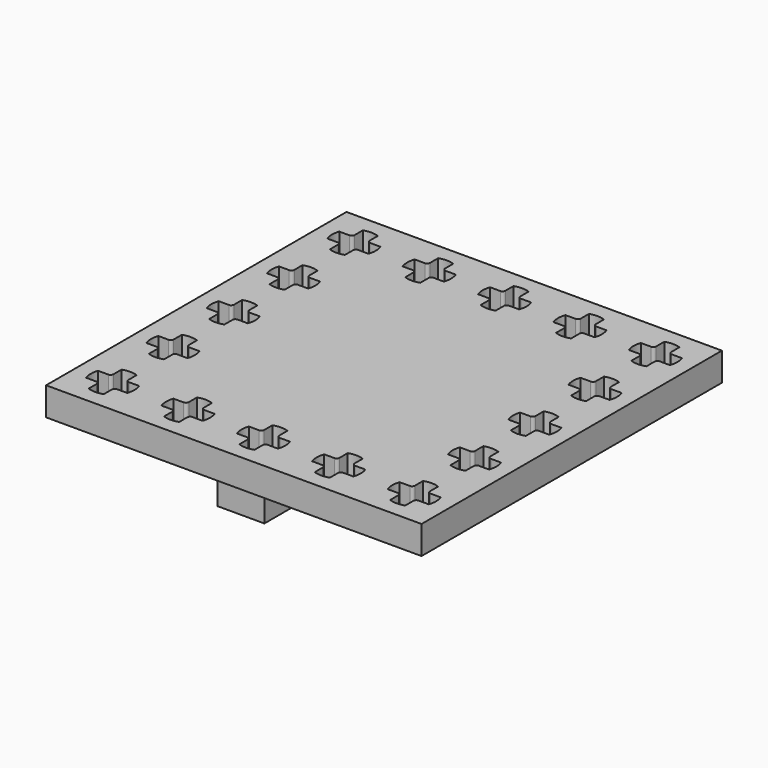
from build123d import *

# Parameters (mm, degrees)
F0_W     = 39.85
F0_H     = 39.85
F1_DEPTH = 6
F3_W     = 39.85
F3_H     = 39.85
F4_DEPTH = 3


# Not quite as in the source:
# - a feature names something its author has since deleted; it is built from what else it names


with BuildPart() as f1:
    # F0 (on Top) → F1 (new body)
    with BuildSketch(Plane.XY):
        Rectangle(F0_W, F0_H)
        with BuildLine():
            ThreePointArc((-16.8, -13.8169688504), (-16, -13.675), (-15.2, -13.8169688504))
            Line((-15.2, -13.8169688504), (-15.2, -14.9))
            ThreePointArc((-15.2, -14.9), (-15.1121320344, -15.1121320344), (-14.9, -15.2))
            Line((-14.9, -15.2), (-13.8169688504, -15.2))
            ThreePointArc((-13.8169688504, -15.2), (-13.675, -16), (-13.8169688504, -16.8))
            Line((-13.8169688504, -16.8), (-14.9, -16.8))
            ThreePointArc((-14.9, -16.8), (-15.1121320344, -16.8878679656), (-15.2, -17.1))
            Line((-15.2, -17.1), (-15.2, -18.1830311496))
            ThreePointArc((-15.2, -18.1830311496), (-16, -18.325), (-16.8, -18.1830311496))
            Line((-16.8, -18.1830311496), (-16.8, -17.1))
            ThreePointArc((-16.8, -17.1), (-16.8878679656, -16.8878679656), (-17.1, -16.8))
            Line((-17.1, -16.8), (-18.1830311496, -16.8))
            ThreePointArc((-18.1830311496, -16.8), (-18.325, -16), (-18.1830311496, -15.2))
            Line((-18.1830311496, -15.2), (-17.1, -15.2))
            ThreePointArc((-17.1, -15.2), (-16.8878679656, -15.1121320344), (-16.8, -14.9))
            Line((-16.8, -14.9), (-16.8, -13.8169688504))
        make_face(mode=Mode.SUBTRACT)
        with BuildLine():
            ThreePointArc((-8.8, -13.8169688504), (-8, -13.675), (-7.2, -13.8169688504))
            Line((-7.2, -13.8169688504), (-7.2, -14.9))
            ThreePointArc((-7.2, -14.9), (-7.1121320344, -15.1121320344), (-6.9, -15.2))
            Line((-6.9, -15.2), (-5.8169688504, -15.2))
            ThreePointArc((-5.8169688504, -15.2), (-5.675, -16), (-5.8169688504, -16.8))
            Line((-5.8169688504, -16.8), (-6.9, -16.8))
            ThreePointArc((-6.9, -16.8), (-7.1121320344, -16.8878679656), (-7.2, -17.1))
            Line((-7.2, -17.1), (-7.2, -18.1830311496))
            ThreePointArc((-7.2, -18.1830311496), (-8, -18.325), (-8.8, -18.1830311496))
            Line((-8.8, -18.1830311496), (-8.8, -17.1))
            ThreePointArc((-8.8, -17.1), (-8.8878679656, -16.8878679656), (-9.1, -16.8))
            Line((-9.1, -16.8), (-10.1830311496, -16.8))
            ThreePointArc((-10.1830311496, -16.8), (-10.325, -16), (-10.1830311496, -15.2))
            Line((-10.1830311496, -15.2), (-9.1, -15.2))
            ThreePointArc((-9.1, -15.2), (-8.8878679656, -15.1121320344), (-8.8, -14.9))
            Line((-8.8, -14.9), (-8.8, -13.8169688504))
        make_face(mode=Mode.SUBTRACT)
        with BuildLine():
            ThreePointArc((-16.8, -5.8169688504), (-16, -5.675), (-15.2, -5.8169688504))
            Line((-15.2, -5.8169688504), (-15.2, -6.9))
            ThreePointArc((-15.2, -6.9), (-15.1121320344, -7.1121320344), (-14.9, -7.2))
            Line((-14.9, -7.2), (-13.8169688504, -7.2))
            ThreePointArc((-13.8169688504, -7.2), (-13.675, -8), (-13.8169688504, -8.8))
            Line((-13.8169688504, -8.8), (-14.9, -8.8))
            ThreePointArc((-14.9, -8.8), (-15.1121320344, -8.8878679656), (-15.2, -9.1))
            Line((-15.2, -9.1), (-15.2, -10.1830311496))
            ThreePointArc((-15.2, -10.1830311496), (-16, -10.325), (-16.8, -10.1830311496))
            Line((-16.8, -10.1830311496), (-16.8, -9.1))
            ThreePointArc((-16.8, -9.1), (-16.8878679656, -8.8878679656), (-17.1, -8.8))
            Line((-17.1, -8.8), (-18.1830311496, -8.8))
            ThreePointArc((-18.1830311496, -8.8), (-18.325, -8), (-18.1830311496, -7.2))
            Line((-18.1830311496, -7.2), (-17.1, -7.2))
            ThreePointArc((-17.1, -7.2), (-16.8878679656, -7.1121320344), (-16.8, -6.9))
            Line((-16.8, -6.9), (-16.8, -5.8169688504))
        make_face(mode=Mode.SUBTRACT)
        with BuildLine():
            ThreePointArc((-8.8, -5.8169688504), (-8, -5.675), (-7.2, -5.8169688504))
            Line((-7.2, -5.8169688504), (-7.2, -6.9))
            ThreePointArc((-7.2, -6.9), (-7.1121320344, -7.1121320344), (-6.9, -7.2))
            Line((-6.9, -7.2), (-5.8169688504, -7.2))
            ThreePointArc((-5.8169688504, -7.2), (-5.675, -8), (-5.8169688504, -8.8))
            Line((-5.8169688504, -8.8), (-6.9, -8.8))
            ThreePointArc((-6.9, -8.8), (-7.1121320344, -8.8878679656), (-7.2, -9.1))
            Line((-7.2, -9.1), (-7.2, -10.1830311496))
            ThreePointArc((-7.2, -10.1830311496), (-8, -10.325), (-8.8, -10.1830311496))
            Line((-8.8, -10.1830311496), (-8.8, -9.1))
            ThreePointArc((-8.8, -9.1), (-8.8878679656, -8.8878679656), (-9.1, -8.8))
            Line((-9.1, -8.8), (-10.1830311496, -8.8))
            ThreePointArc((-10.1830311496, -8.8), (-10.325, -8), (-10.1830311496, -7.2))
            Line((-10.1830311496, -7.2), (-9.1, -7.2))
            ThreePointArc((-9.1, -7.2), (-8.8878679656, -7.1121320344), (-8.8, -6.9))
            Line((-8.8, -6.9), (-8.8, -5.8169688504))
        make_face(mode=Mode.SUBTRACT)
        with BuildLine():
            ThreePointArc((-0.8, -13.8169688504), (0, -13.675), (0.8, -13.8169688504))
            Line((0.8, -13.8169688504), (0.8, -14.9))
            ThreePointArc((0.8, -14.9), (0.8878679656, -15.1121320344), (1.1, -15.2))
            Line((1.1, -15.2), (2.1830311496, -15.2))
            ThreePointArc((2.1830311496, -15.2), (2.325, -16), (2.1830311496, -16.8))
            Line((2.1830311496, -16.8), (1.1, -16.8))
            ThreePointArc((1.1, -16.8), (0.8878679656, -16.8878679656), (0.8, -17.1))
            Line((0.8, -17.1), (0.8, -18.1830311496))
            ThreePointArc((0.8, -18.1830311496), (0, -18.325), (-0.8, -18.1830311496))
            Line((-0.8, -18.1830311496), (-0.8, -17.1))
            ThreePointArc((-0.8, -17.1), (-0.8878679656, -16.8878679656), (-1.1, -16.8))
            Line((-1.1, -16.8), (-2.1830311496, -16.8))
            ThreePointArc((-2.1830311496, -16.8), (-2.325, -16), (-2.1830311496, -15.2))
            Line((-2.1830311496, -15.2), (-1.1, -15.2))
            ThreePointArc((-1.1, -15.2), (-0.8878679656, -15.1121320344), (-0.8, -14.9))
            Line((-0.8, -14.9), (-0.8, -13.8169688504))
        make_face(mode=Mode.SUBTRACT)
        with BuildLine():
            ThreePointArc((7.2, -13.8169688504), (8, -13.675), (8.8, -13.8169688504))
            Line((8.8, -13.8169688504), (8.8, -14.9))
            ThreePointArc((8.8, -14.9), (8.8878679656, -15.1121320344), (9.1, -15.2))
            Line((9.1, -15.2), (10.1830311496, -15.2))
            ThreePointArc((10.1830311496, -15.2), (10.325, -16), (10.1830311496, -16.8))
            Line((10.1830311496, -16.8), (9.1, -16.8))
            ThreePointArc((9.1, -16.8), (8.8878679656, -16.8878679656), (8.8, -17.1))
            Line((8.8, -17.1), (8.8, -18.1830311496))
            ThreePointArc((8.8, -18.1830311496), (8, -18.325), (7.2, -18.1830311496))
            Line((7.2, -18.1830311496), (7.2, -17.1))
            ThreePointArc((7.2, -17.1), (7.1121320344, -16.8878679656), (6.9, -16.8))
            Line((6.9, -16.8), (5.8169688504, -16.8))
            ThreePointArc((5.8169688504, -16.8), (5.675, -16), (5.8169688504, -15.2))
            Line((5.8169688504, -15.2), (6.9, -15.2))
            ThreePointArc((6.9, -15.2), (7.1121320344, -15.1121320344), (7.2, -14.9))
            Line((7.2, -14.9), (7.2, -13.8169688504))
        make_face(mode=Mode.SUBTRACT)
        with BuildLine():
            ThreePointArc((15.2, -13.8169688504), (16, -13.675), (16.8, -13.8169688504))
            Line((16.8, -13.8169688504), (16.8, -14.9))
            ThreePointArc((16.8, -14.9), (16.8878679656, -15.1121320344), (17.1, -15.2))
            Line((17.1, -15.2), (18.1830311496, -15.2))
            ThreePointArc((18.1830311496, -15.2), (18.325, -16), (18.1830311496, -16.8))
            Line((18.1830311496, -16.8), (17.1, -16.8))
            ThreePointArc((17.1, -16.8), (16.8878679656, -16.8878679656), (16.8, -17.1))
            Line((16.8, -17.1), (16.8, -18.1830311496))
            ThreePointArc((16.8, -18.1830311496), (16, -18.325), (15.2, -18.1830311496))
            Line((15.2, -18.1830311496), (15.2, -17.1))
            ThreePointArc((15.2, -17.1), (15.1121320344, -16.8878679656), (14.9, -16.8))
            Line((14.9, -16.8), (13.8169688504, -16.8))
            ThreePointArc((13.8169688504, -16.8), (13.675, -16), (13.8169688504, -15.2))
            Line((13.8169688504, -15.2), (14.9, -15.2))
            ThreePointArc((14.9, -15.2), (15.1121320344, -15.1121320344), (15.2, -14.9))
            Line((15.2, -14.9), (15.2, -13.8169688504))
        make_face(mode=Mode.SUBTRACT)
        with BuildLine():
            ThreePointArc((-0.8, -5.8169688504), (0, -5.675), (0.8, -5.8169688504))
            Line((0.8, -5.8169688504), (0.8, -6.9))
            ThreePointArc((0.8, -6.9), (0.8878679656, -7.1121320344), (1.1, -7.2))
            Line((1.1, -7.2), (2.1830311496, -7.2))
            ThreePointArc((2.1830311496, -7.2), (2.325, -8), (2.1830311496, -8.8))
            Line((2.1830311496, -8.8), (1.1, -8.8))
            ThreePointArc((1.1, -8.8), (0.8878679656, -8.8878679656), (0.8, -9.1))
            Line((0.8, -9.1), (0.8, -10.1830311496))
            ThreePointArc((0.8, -10.1830311496), (0, -10.325), (-0.8, -10.1830311496))
            Line((-0.8, -10.1830311496), (-0.8, -9.1))
            ThreePointArc((-0.8, -9.1), (-0.8878679656, -8.8878679656), (-1.1, -8.8))
            Line((-1.1, -8.8), (-2.1830311496, -8.8))
            ThreePointArc((-2.1830311496, -8.8), (-2.325, -8), (-2.1830311496, -7.2))
            Line((-2.1830311496, -7.2), (-1.1, -7.2))
            ThreePointArc((-1.1, -7.2), (-0.8878679656, -7.1121320344), (-0.8, -6.9))
            Line((-0.8, -6.9), (-0.8, -5.8169688504))
        make_face(mode=Mode.SUBTRACT)
        with BuildLine():
            ThreePointArc((7.2, -5.8169688504), (8, -5.675), (8.8, -5.8169688504))
            Line((8.8, -5.8169688504), (8.8, -6.9))
            ThreePointArc((8.8, -6.9), (8.8878679656, -7.1121320344), (9.1, -7.2))
            Line((9.1, -7.2), (10.1830311496, -7.2))
            ThreePointArc((10.1830311496, -7.2), (10.325, -8), (10.1830311496, -8.8))
            Line((10.1830311496, -8.8), (9.1, -8.8))
            ThreePointArc((9.1, -8.8), (8.8878679656, -8.8878679656), (8.8, -9.1))
            Line((8.8, -9.1), (8.8, -10.1830311496))
            ThreePointArc((8.8, -10.1830311496), (8, -10.325), (7.2, -10.1830311496))
            Line((7.2, -10.1830311496), (7.2, -9.1))
            ThreePointArc((7.2, -9.1), (7.1121320344, -8.8878679656), (6.9, -8.8))
            Line((6.9, -8.8), (5.8169688504, -8.8))
            ThreePointArc((5.8169688504, -8.8), (5.675, -8), (5.8169688504, -7.2))
            Line((5.8169688504, -7.2), (6.9, -7.2))
            ThreePointArc((6.9, -7.2), (7.1121320344, -7.1121320344), (7.2, -6.9))
            Line((7.2, -6.9), (7.2, -5.8169688504))
        make_face(mode=Mode.SUBTRACT)
        with BuildLine():
            ThreePointArc((15.2, -5.8169688504), (16, -5.675), (16.8, -5.8169688504))
            Line((16.8, -5.8169688504), (16.8, -6.9))
            ThreePointArc((16.8, -6.9), (16.8878679656, -7.1121320344), (17.1, -7.2))
            Line((17.1, -7.2), (18.1830311496, -7.2))
            ThreePointArc((18.1830311496, -7.2), (18.325, -8), (18.1830311496, -8.8))
            Line((18.1830311496, -8.8), (17.1, -8.8))
            ThreePointArc((17.1, -8.8), (16.8878679656, -8.8878679656), (16.8, -9.1))
            Line((16.8, -9.1), (16.8, -10.1830311496))
            ThreePointArc((16.8, -10.1830311496), (16, -10.325), (15.2, -10.1830311496))
            Line((15.2, -10.1830311496), (15.2, -9.1))
            ThreePointArc((15.2, -9.1), (15.1121320344, -8.8878679656), (14.9, -8.8))
            Line((14.9, -8.8), (13.8169688504, -8.8))
            ThreePointArc((13.8169688504, -8.8), (13.675, -8), (13.8169688504, -7.2))
            Line((13.8169688504, -7.2), (14.9, -7.2))
            ThreePointArc((14.9, -7.2), (15.1121320344, -7.1121320344), (15.2, -6.9))
            Line((15.2, -6.9), (15.2, -5.8169688504))
        make_face(mode=Mode.SUBTRACT)
        with BuildLine():
            ThreePointArc((-16.8, 2.1830311496), (-16, 2.325), (-15.2, 2.1830311496))
            Line((-15.2, 2.1830311496), (-15.2, 1.1))
            ThreePointArc((-15.2, 1.1), (-15.1121320344, 0.8878679656), (-14.9, 0.8))
            Line((-14.9, 0.8), (-13.8169688504, 0.8))
            ThreePointArc((-13.8169688504, 0.8), (-13.675, 0), (-13.8169688504, -0.8))
            Line((-13.8169688504, -0.8), (-14.9, -0.8))
            ThreePointArc((-14.9, -0.8), (-15.1121320344, -0.8878679656), (-15.2, -1.1))
            Line((-15.2, -1.1), (-15.2, -2.1830311496))
            ThreePointArc((-15.2, -2.1830311496), (-16, -2.325), (-16.8, -2.1830311496))
            Line((-16.8, -2.1830311496), (-16.8, -1.1))
            ThreePointArc((-16.8, -1.1), (-16.8878679656, -0.8878679656), (-17.1, -0.8))
            Line((-17.1, -0.8), (-18.1830311496, -0.8))
            ThreePointArc((-18.1830311496, -0.8), (-18.325, 0), (-18.1830311496, 0.8))
            Line((-18.1830311496, 0.8), (-17.1, 0.8))
            ThreePointArc((-17.1, 0.8), (-16.8878679656, 0.8878679656), (-16.8, 1.1))
            Line((-16.8, 1.1), (-16.8, 2.1830311496))
        make_face(mode=Mode.SUBTRACT)
        with BuildLine():
            ThreePointArc((-16.8, 10.1830311496), (-16, 10.325), (-15.2, 10.1830311496))
            Line((-15.2, 10.1830311496), (-15.2, 9.1))
            ThreePointArc((-15.2, 9.1), (-15.1121320344, 8.8878679656), (-14.9, 8.8))
            Line((-14.9, 8.8), (-13.8169688504, 8.8))
            ThreePointArc((-13.8169688504, 8.8), (-13.675, 8), (-13.8169688504, 7.2))
            Line((-13.8169688504, 7.2), (-14.9, 7.2))
            ThreePointArc((-14.9, 7.2), (-15.1121320344, 7.1121320344), (-15.2, 6.9))
            Line((-15.2, 6.9), (-15.2, 5.8169688504))
            ThreePointArc((-15.2, 5.8169688504), (-16, 5.675), (-16.8, 5.8169688504))
            Line((-16.8, 5.8169688504), (-16.8, 6.9))
            ThreePointArc((-16.8, 6.9), (-16.8878679656, 7.1121320344), (-17.1, 7.2))
            Line((-17.1, 7.2), (-18.1830311496, 7.2))
            ThreePointArc((-18.1830311496, 7.2), (-18.325, 8), (-18.1830311496, 8.8))
            Line((-18.1830311496, 8.8), (-17.1, 8.8))
            ThreePointArc((-17.1, 8.8), (-16.8878679656, 8.8878679656), (-16.8, 9.1))
            Line((-16.8, 9.1), (-16.8, 10.1830311496))
        make_face(mode=Mode.SUBTRACT)
        with BuildLine():
            ThreePointArc((-8.8, 2.1830311496), (-8, 2.325), (-7.2, 2.1830311496))
            Line((-7.2, 2.1830311496), (-7.2, 1.1))
            ThreePointArc((-7.2, 1.1), (-7.1121320344, 0.8878679656), (-6.9, 0.8))
            Line((-6.9, 0.8), (-5.8169688504, 0.8))
            ThreePointArc((-5.8169688504, 0.8), (-5.675, 0), (-5.8169688504, -0.8))
            Line((-5.8169688504, -0.8), (-6.9, -0.8))
            ThreePointArc((-6.9, -0.8), (-7.1121320344, -0.8878679656), (-7.2, -1.1))
            Line((-7.2, -1.1), (-7.2, -2.1830311496))
            ThreePointArc((-7.2, -2.1830311496), (-8, -2.325), (-8.8, -2.1830311496))
            Line((-8.8, -2.1830311496), (-8.8, -1.1))
            ThreePointArc((-8.8, -1.1), (-8.8878679656, -0.8878679656), (-9.1, -0.8))
            Line((-9.1, -0.8), (-10.1830311496, -0.8))
            ThreePointArc((-10.1830311496, -0.8), (-10.325, 0), (-10.1830311496, 0.8))
            Line((-10.1830311496, 0.8), (-9.1, 0.8))
            ThreePointArc((-9.1, 0.8), (-8.8878679656, 0.8878679656), (-8.8, 1.1))
            Line((-8.8, 1.1), (-8.8, 2.1830311496))
        make_face(mode=Mode.SUBTRACT)
        with BuildLine():
            ThreePointArc((-8.8, 10.1830311496), (-8, 10.325), (-7.2, 10.1830311496))
            Line((-7.2, 10.1830311496), (-7.2, 9.1))
            ThreePointArc((-7.2, 9.1), (-7.1121320344, 8.8878679656), (-6.9, 8.8))
            Line((-6.9, 8.8), (-5.8169688504, 8.8))
            ThreePointArc((-5.8169688504, 8.8), (-5.675, 8), (-5.8169688504, 7.2))
            Line((-5.8169688504, 7.2), (-6.9, 7.2))
            ThreePointArc((-6.9, 7.2), (-7.1121320344, 7.1121320344), (-7.2, 6.9))
            Line((-7.2, 6.9), (-7.2, 5.8169688504))
            ThreePointArc((-7.2, 5.8169688504), (-8, 5.675), (-8.8, 5.8169688504))
            Line((-8.8, 5.8169688504), (-8.8, 6.9))
            ThreePointArc((-8.8, 6.9), (-8.8878679656, 7.1121320344), (-9.1, 7.2))
            Line((-9.1, 7.2), (-10.1830311496, 7.2))
            ThreePointArc((-10.1830311496, 7.2), (-10.325, 8), (-10.1830311496, 8.8))
            Line((-10.1830311496, 8.8), (-9.1, 8.8))
            ThreePointArc((-9.1, 8.8), (-8.8878679656, 8.8878679656), (-8.8, 9.1))
            Line((-8.8, 9.1), (-8.8, 10.1830311496))
        make_face(mode=Mode.SUBTRACT)
        with BuildLine():
            ThreePointArc((-16.8, 18.1830311496), (-16, 18.325), (-15.2, 18.1830311496))
            Line((-15.2, 18.1830311496), (-15.2, 17.1))
            ThreePointArc((-15.2, 17.1), (-15.1121320344, 16.8878679656), (-14.9, 16.8))
            Line((-14.9, 16.8), (-13.8169688504, 16.8))
            ThreePointArc((-13.8169688504, 16.8), (-13.675, 16), (-13.8169688504, 15.2))
            Line((-13.8169688504, 15.2), (-14.9, 15.2))
            ThreePointArc((-14.9, 15.2), (-15.1121320344, 15.1121320344), (-15.2, 14.9))
            Line((-15.2, 14.9), (-15.2, 13.8169688504))
            ThreePointArc((-15.2, 13.8169688504), (-16, 13.675), (-16.8, 13.8169688504))
            Line((-16.8, 13.8169688504), (-16.8, 14.9))
            ThreePointArc((-16.8, 14.9), (-16.8878679656, 15.1121320344), (-17.1, 15.2))
            Line((-17.1, 15.2), (-18.1830311496, 15.2))
            ThreePointArc((-18.1830311496, 15.2), (-18.325, 16), (-18.1830311496, 16.8))
            Line((-18.1830311496, 16.8), (-17.1, 16.8))
            ThreePointArc((-17.1, 16.8), (-16.8878679656, 16.8878679656), (-16.8, 17.1))
            Line((-16.8, 17.1), (-16.8, 18.1830311496))
        make_face(mode=Mode.SUBTRACT)
        with BuildLine():
            ThreePointArc((-8.8, 18.1830311496), (-8, 18.325), (-7.2, 18.1830311496))
            Line((-7.2, 18.1830311496), (-7.2, 17.1))
            ThreePointArc((-7.2, 17.1), (-7.1121320344, 16.8878679656), (-6.9, 16.8))
            Line((-6.9, 16.8), (-5.8169688504, 16.8))
            ThreePointArc((-5.8169688504, 16.8), (-5.675, 16), (-5.8169688504, 15.2))
            Line((-5.8169688504, 15.2), (-6.9, 15.2))
            ThreePointArc((-6.9, 15.2), (-7.1121320344, 15.1121320344), (-7.2, 14.9))
            Line((-7.2, 14.9), (-7.2, 13.8169688504))
            ThreePointArc((-7.2, 13.8169688504), (-8, 13.675), (-8.8, 13.8169688504))
            Line((-8.8, 13.8169688504), (-8.8, 14.9))
            ThreePointArc((-8.8, 14.9), (-8.8878679656, 15.1121320344), (-9.1, 15.2))
            Line((-9.1, 15.2), (-10.1830311496, 15.2))
            ThreePointArc((-10.1830311496, 15.2), (-10.325, 16), (-10.1830311496, 16.8))
            Line((-10.1830311496, 16.8), (-9.1, 16.8))
            ThreePointArc((-9.1, 16.8), (-8.8878679656, 16.8878679656), (-8.8, 17.1))
            Line((-8.8, 17.1), (-8.8, 18.1830311496))
        make_face(mode=Mode.SUBTRACT)
        with BuildLine():
            ThreePointArc((-0.8, 2.1830311496), (0, 2.325), (0.8, 2.1830311496))
            Line((0.8, 2.1830311496), (0.8, 1.1))
            ThreePointArc((0.8, 1.1), (0.8878679656, 0.8878679656), (1.1, 0.8))
            Line((1.1, 0.8), (2.1830311496, 0.8))
            ThreePointArc((2.1830311496, 0.8), (2.325, 0), (2.1830311496, -0.8))
            Line((2.1830311496, -0.8), (1.1, -0.8))
            ThreePointArc((1.1, -0.8), (0.8878679656, -0.8878679656), (0.8, -1.1))
            Line((0.8, -1.1), (0.8, -2.1830311496))
            ThreePointArc((0.8, -2.1830311496), (0, -2.325), (-0.8, -2.1830311496))
            Line((-0.8, -2.1830311496), (-0.8, -1.1))
            ThreePointArc((-0.8, -1.1), (-0.8878679656, -0.8878679656), (-1.1, -0.8))
            Line((-1.1, -0.8), (-2.1830311496, -0.8))
            ThreePointArc((-2.1830311496, -0.8), (-2.325, 0), (-2.1830311496, 0.8))
            Line((-2.1830311496, 0.8), (-1.1, 0.8))
            ThreePointArc((-1.1, 0.8), (-0.8878679656, 0.8878679656), (-0.8, 1.1))
            Line((-0.8, 1.1), (-0.8, 2.1830311496))
        make_face(mode=Mode.SUBTRACT)
        with BuildLine():
            ThreePointArc((7.2, 2.1830311496), (8, 2.325), (8.8, 2.1830311496))
            Line((8.8, 2.1830311496), (8.8, 1.1))
            ThreePointArc((8.8, 1.1), (8.8878679656, 0.8878679656), (9.1, 0.8))
            Line((9.1, 0.8), (10.1830311496, 0.8))
            ThreePointArc((10.1830311496, 0.8), (10.325, 0), (10.1830311496, -0.8))
            Line((10.1830311496, -0.8), (9.1, -0.8))
            ThreePointArc((9.1, -0.8), (8.8878679656, -0.8878679656), (8.8, -1.1))
            Line((8.8, -1.1), (8.8, -2.1830311496))
            ThreePointArc((8.8, -2.1830311496), (8, -2.325), (7.2, -2.1830311496))
            Line((7.2, -2.1830311496), (7.2, -1.1))
            ThreePointArc((7.2, -1.1), (7.1121320344, -0.8878679656), (6.9, -0.8))
            Line((6.9, -0.8), (5.8169688504, -0.8))
            ThreePointArc((5.8169688504, -0.8), (5.675, 0), (5.8169688504, 0.8))
            Line((5.8169688504, 0.8), (6.9, 0.8))
            ThreePointArc((6.9, 0.8), (7.1121320344, 0.8878679656), (7.2, 1.1))
            Line((7.2, 1.1), (7.2, 2.1830311496))
        make_face(mode=Mode.SUBTRACT)
        with BuildLine():
            ThreePointArc((-0.8, 10.1830311496), (0, 10.325), (0.8, 10.1830311496))
            Line((0.8, 10.1830311496), (0.8, 9.1))
            ThreePointArc((0.8, 9.1), (0.8878679656, 8.8878679656), (1.1, 8.8))
            Line((1.1, 8.8), (2.1830311496, 8.8))
            ThreePointArc((2.1830311496, 8.8), (2.325, 8), (2.1830311496, 7.2))
            Line((2.1830311496, 7.2), (1.1, 7.2))
            ThreePointArc((1.1, 7.2), (0.8878679656, 7.1121320344), (0.8, 6.9))
            Line((0.8, 6.9), (0.8, 5.8169688504))
            ThreePointArc((0.8, 5.8169688504), (0, 5.675), (-0.8, 5.8169688504))
            Line((-0.8, 5.8169688504), (-0.8, 6.9))
            ThreePointArc((-0.8, 6.9), (-0.8878679656, 7.1121320344), (-1.1, 7.2))
            Line((-1.1, 7.2), (-2.1830311496, 7.2))
            ThreePointArc((-2.1830311496, 7.2), (-2.325, 8), (-2.1830311496, 8.8))
            Line((-2.1830311496, 8.8), (-1.1, 8.8))
            ThreePointArc((-1.1, 8.8), (-0.8878679656, 8.8878679656), (-0.8, 9.1))
            Line((-0.8, 9.1), (-0.8, 10.1830311496))
        make_face(mode=Mode.SUBTRACT)
        with BuildLine():
            ThreePointArc((7.2, 10.1830311496), (8, 10.325), (8.8, 10.1830311496))
            Line((8.8, 10.1830311496), (8.8, 9.1))
            ThreePointArc((8.8, 9.1), (8.8878679656, 8.8878679656), (9.1, 8.8))
            Line((9.1, 8.8), (10.1830311496, 8.8))
            ThreePointArc((10.1830311496, 8.8), (10.325, 8), (10.1830311496, 7.2))
            Line((10.1830311496, 7.2), (9.1, 7.2))
            ThreePointArc((9.1, 7.2), (8.8878679656, 7.1121320344), (8.8, 6.9))
            Line((8.8, 6.9), (8.8, 5.8169688504))
            ThreePointArc((8.8, 5.8169688504), (8, 5.675), (7.2, 5.8169688504))
            Line((7.2, 5.8169688504), (7.2, 6.9))
            ThreePointArc((7.2, 6.9), (7.1121320344, 7.1121320344), (6.9, 7.2))
            Line((6.9, 7.2), (5.8169688504, 7.2))
            ThreePointArc((5.8169688504, 7.2), (5.675, 8), (5.8169688504, 8.8))
            Line((5.8169688504, 8.8), (6.9, 8.8))
            ThreePointArc((6.9, 8.8), (7.1121320344, 8.8878679656), (7.2, 9.1))
            Line((7.2, 9.1), (7.2, 10.1830311496))
        make_face(mode=Mode.SUBTRACT)
        with BuildLine():
            ThreePointArc((15.2, 2.1830311496), (16, 2.325), (16.8, 2.1830311496))
            Line((16.8, 2.1830311496), (16.8, 1.1))
            ThreePointArc((16.8, 1.1), (16.8878679656, 0.8878679656), (17.1, 0.8))
            Line((17.1, 0.8), (18.1830311496, 0.8))
            ThreePointArc((18.1830311496, 0.8), (18.325, 0), (18.1830311496, -0.8))
            Line((18.1830311496, -0.8), (17.1, -0.8))
            ThreePointArc((17.1, -0.8), (16.8878679656, -0.8878679656), (16.8, -1.1))
            Line((16.8, -1.1), (16.8, -2.1830311496))
            ThreePointArc((16.8, -2.1830311496), (16, -2.325), (15.2, -2.1830311496))
            Line((15.2, -2.1830311496), (15.2, -1.1))
            ThreePointArc((15.2, -1.1), (15.1121320344, -0.8878679656), (14.9, -0.8))
            Line((14.9, -0.8), (13.8169688504, -0.8))
            ThreePointArc((13.8169688504, -0.8), (13.675, 0), (13.8169688504, 0.8))
            Line((13.8169688504, 0.8), (14.9, 0.8))
            ThreePointArc((14.9, 0.8), (15.1121320344, 0.8878679656), (15.2, 1.1))
            Line((15.2, 1.1), (15.2, 2.1830311496))
        make_face(mode=Mode.SUBTRACT)
        with BuildLine():
            ThreePointArc((15.2, 10.1830311496), (16, 10.325), (16.8, 10.1830311496))
            Line((16.8, 10.1830311496), (16.8, 9.1))
            ThreePointArc((16.8, 9.1), (16.8878679656, 8.8878679656), (17.1, 8.8))
            Line((17.1, 8.8), (18.1830311496, 8.8))
            ThreePointArc((18.1830311496, 8.8), (18.325, 8), (18.1830311496, 7.2))
            Line((18.1830311496, 7.2), (17.1, 7.2))
            ThreePointArc((17.1, 7.2), (16.8878679656, 7.1121320344), (16.8, 6.9))
            Line((16.8, 6.9), (16.8, 5.8169688504))
            ThreePointArc((16.8, 5.8169688504), (16, 5.675), (15.2, 5.8169688504))
            Line((15.2, 5.8169688504), (15.2, 6.9))
            ThreePointArc((15.2, 6.9), (15.1121320344, 7.1121320344), (14.9, 7.2))
            Line((14.9, 7.2), (13.8169688504, 7.2))
            ThreePointArc((13.8169688504, 7.2), (13.675, 8), (13.8169688504, 8.8))
            Line((13.8169688504, 8.8), (14.9, 8.8))
            ThreePointArc((14.9, 8.8), (15.1121320344, 8.8878679656), (15.2, 9.1))
            Line((15.2, 9.1), (15.2, 10.1830311496))
        make_face(mode=Mode.SUBTRACT)
        with BuildLine():
            ThreePointArc((-0.8, 18.1830311496), (0, 18.325), (0.8, 18.1830311496))
            Line((0.8, 18.1830311496), (0.8, 17.1))
            ThreePointArc((0.8, 17.1), (0.8878679656, 16.8878679656), (1.1, 16.8))
            Line((1.1, 16.8), (2.1830311496, 16.8))
            ThreePointArc((2.1830311496, 16.8), (2.325, 16), (2.1830311496, 15.2))
            Line((2.1830311496, 15.2), (1.1, 15.2))
            ThreePointArc((1.1, 15.2), (0.8878679656, 15.1121320344), (0.8, 14.9))
            Line((0.8, 14.9), (0.8, 13.8169688504))
            ThreePointArc((0.8, 13.8169688504), (0, 13.675), (-0.8, 13.8169688504))
            Line((-0.8, 13.8169688504), (-0.8, 14.9))
            ThreePointArc((-0.8, 14.9), (-0.8878679656, 15.1121320344), (-1.1, 15.2))
            Line((-1.1, 15.2), (-2.1830311496, 15.2))
            ThreePointArc((-2.1830311496, 15.2), (-2.325, 16), (-2.1830311496, 16.8))
            Line((-2.1830311496, 16.8), (-1.1, 16.8))
            ThreePointArc((-1.1, 16.8), (-0.8878679656, 16.8878679656), (-0.8, 17.1))
            Line((-0.8, 17.1), (-0.8, 18.1830311496))
        make_face(mode=Mode.SUBTRACT)
        with BuildLine():
            ThreePointArc((7.2, 18.1830311496), (8, 18.325), (8.8, 18.1830311496))
            Line((8.8, 18.1830311496), (8.8, 17.1))
            ThreePointArc((8.8, 17.1), (8.8878679656, 16.8878679656), (9.1, 16.8))
            Line((9.1, 16.8), (10.1830311496, 16.8))
            ThreePointArc((10.1830311496, 16.8), (10.325, 16), (10.1830311496, 15.2))
            Line((10.1830311496, 15.2), (9.1, 15.2))
            ThreePointArc((9.1, 15.2), (8.8878679656, 15.1121320344), (8.8, 14.9))
            Line((8.8, 14.9), (8.8, 13.8169688504))
            ThreePointArc((8.8, 13.8169688504), (8, 13.675), (7.2, 13.8169688504))
            Line((7.2, 13.8169688504), (7.2, 14.9))
            ThreePointArc((7.2, 14.9), (7.1121320344, 15.1121320344), (6.9, 15.2))
            Line((6.9, 15.2), (5.8169688504, 15.2))
            ThreePointArc((5.8169688504, 15.2), (5.675, 16), (5.8169688504, 16.8))
            Line((5.8169688504, 16.8), (6.9, 16.8))
            ThreePointArc((6.9, 16.8), (7.1121320344, 16.8878679656), (7.2, 17.1))
            Line((7.2, 17.1), (7.2, 18.1830311496))
        make_face(mode=Mode.SUBTRACT)
        with BuildLine():
            ThreePointArc((15.2, 18.1830311496), (16, 18.325), (16.8, 18.1830311496))
            Line((16.8, 18.1830311496), (16.8, 17.1))
            ThreePointArc((16.8, 17.1), (16.8878679656, 16.8878679656), (17.1, 16.8))
            Line((17.1, 16.8), (18.1830311496, 16.8))
            ThreePointArc((18.1830311496, 16.8), (18.325, 16), (18.1830311496, 15.2))
            Line((18.1830311496, 15.2), (17.1, 15.2))
            ThreePointArc((17.1, 15.2), (16.8878679656, 15.1121320344), (16.8, 14.9))
            Line((16.8, 14.9), (16.8, 13.8169688504))
            ThreePointArc((16.8, 13.8169688504), (16, 13.675), (15.2, 13.8169688504))
            Line((15.2, 13.8169688504), (15.2, 14.9))
            ThreePointArc((15.2, 14.9), (15.1121320344, 15.1121320344), (14.9, 15.2))
            Line((14.9, 15.2), (13.8169688504, 15.2))
            ThreePointArc((13.8169688504, 15.2), (13.675, 16), (13.8169688504, 16.8))
            Line((13.8169688504, 16.8), (14.9, 16.8))
            ThreePointArc((14.9, 16.8), (15.1121320344, 16.8878679656), (15.2, 17.1))
            Line((15.2, 17.1), (15.2, 18.1830311496))
        make_face(mode=Mode.SUBTRACT)
        with BuildLine():
            Line((8.8, 9.1), (8.8, 10.1830311496))
            ThreePointArc((8.8, 10.1830311496), (8, 10.325), (7.2, 10.1830311496))
            Line((7.2, 10.1830311496), (7.2, 9.1))
            ThreePointArc((7.2, 9.1), (7.1121320344, 8.8878679656), (6.9, 8.8))
            Line((6.9, 8.8), (5.8169688504, 8.8))
            ThreePointArc((5.8169688504, 8.8), (5.675, 8), (5.8169688504, 7.2))
            Line((5.8169688504, 7.2), (6.9, 7.2))
            ThreePointArc((6.9, 7.2), (7.1121320344, 7.1121320344), (7.2, 6.9))
            Line((7.2, 6.9), (7.2, 5.8169688504))
            ThreePointArc((7.2, 5.8169688504), (8, 5.675), (8.8, 5.8169688504))
            Line((8.8, 5.8169688504), (8.8, 6.9))
            ThreePointArc((8.8, 6.9), (8.8878679656, 7.1121320344), (9.1, 7.2))
            Line((9.1, 7.2), (10.1830311496, 7.2))
            ThreePointArc((10.1830311496, 7.2), (10.325, 8), (10.1830311496, 8.8))
            Line((10.1830311496, 8.8), (9.1, 8.8))
            ThreePointArc((9.1, 8.8), (8.8878679656, 8.8878679656), (8.8, 9.1))
        make_face()
        with BuildLine():
            Line((8.8, 1.1), (8.8, 2.1830311496))
            ThreePointArc((8.8, 2.1830311496), (8, 2.325), (7.2, 2.1830311496))
            Line((7.2, 2.1830311496), (7.2, 1.1))
            ThreePointArc((7.2, 1.1), (7.1121320344, 0.8878679656), (6.9, 0.8))
            Line((6.9, 0.8), (5.8169688504, 0.8))
            ThreePointArc((5.8169688504, 0.8), (5.675, 0), (5.8169688504, -0.8))
            Line((5.8169688504, -0.8), (6.9, -0.8))
            ThreePointArc((6.9, -0.8), (7.1121320344, -0.8878679656), (7.2, -1.1))
            Line((7.2, -1.1), (7.2, -2.1830311496))
            ThreePointArc((7.2, -2.1830311496), (8, -2.325), (8.8, -2.1830311496))
            Line((8.8, -2.1830311496), (8.8, -1.1))
            ThreePointArc((8.8, -1.1), (8.8878679656, -0.8878679656), (9.1, -0.8))
            Line((9.1, -0.8), (10.1830311496, -0.8))
            ThreePointArc((10.1830311496, -0.8), (10.325, 0), (10.1830311496, 0.8))
            Line((10.1830311496, 0.8), (9.1, 0.8))
            ThreePointArc((9.1, 0.8), (8.8878679656, 0.8878679656), (8.8, 1.1))
        make_face()
        with BuildLine():
            Line((8.8, -6.9), (8.8, -5.8169688504))
            ThreePointArc((8.8, -5.8169688504), (8, -5.675), (7.2, -5.8169688504))
            Line((7.2, -5.8169688504), (7.2, -6.9))
            ThreePointArc((7.2, -6.9), (7.1121320344, -7.1121320344), (6.9, -7.2))
            Line((6.9, -7.2), (5.8169688504, -7.2))
            ThreePointArc((5.8169688504, -7.2), (5.675, -8), (5.8169688504, -8.8))
            Line((5.8169688504, -8.8), (6.9, -8.8))
            ThreePointArc((6.9, -8.8), (7.1121320344, -8.8878679656), (7.2, -9.1))
            Line((7.2, -9.1), (7.2, -10.1830311496))
            ThreePointArc((7.2, -10.1830311496), (8, -10.325), (8.8, -10.1830311496))
            Line((8.8, -10.1830311496), (8.8, -9.1))
            ThreePointArc((8.8, -9.1), (8.8878679656, -8.8878679656), (9.1, -8.8))
            Line((9.1, -8.8), (10.1830311496, -8.8))
            ThreePointArc((10.1830311496, -8.8), (10.325, -8), (10.1830311496, -7.2))
            Line((10.1830311496, -7.2), (9.1, -7.2))
            ThreePointArc((9.1, -7.2), (8.8878679656, -7.1121320344), (8.8, -6.9))
        make_face()
        with BuildLine():
            Line((-7.2, 1.1), (-7.2, 2.1830311496))
            ThreePointArc((-7.2, 2.1830311496), (-8, 2.325), (-8.8, 2.1830311496))
            Line((-8.8, 2.1830311496), (-8.8, 1.1))
            ThreePointArc((-8.8, 1.1), (-8.8878679656, 0.8878679656), (-9.1, 0.8))
            Line((-9.1, 0.8), (-10.1830311496, 0.8))
            ThreePointArc((-10.1830311496, 0.8), (-10.325, 0), (-10.1830311496, -0.8))
            Line((-10.1830311496, -0.8), (-9.1, -0.8))
            ThreePointArc((-9.1, -0.8), (-8.8878679656, -0.8878679656), (-8.8, -1.1))
            Line((-8.8, -1.1), (-8.8, -2.1830311496))
            ThreePointArc((-8.8, -2.1830311496), (-8, -2.325), (-7.2, -2.1830311496))
            Line((-7.2, -2.1830311496), (-7.2, -1.1))
            ThreePointArc((-7.2, -1.1), (-7.1121320344, -0.8878679656), (-6.9, -0.8))
            Line((-6.9, -0.8), (-5.8169688504, -0.8))
            ThreePointArc((-5.8169688504, -0.8), (-5.675, 0), (-5.8169688504, 0.8))
            Line((-5.8169688504, 0.8), (-6.9, 0.8))
            ThreePointArc((-6.9, 0.8), (-7.1121320344, 0.8878679656), (-7.2, 1.1))
        make_face()
        with BuildLine():
            Line((-7.2, -6.9), (-7.2, -5.8169688504))
            ThreePointArc((-7.2, -5.8169688504), (-8, -5.675), (-8.8, -5.8169688504))
            Line((-8.8, -5.8169688504), (-8.8, -6.9))
            ThreePointArc((-8.8, -6.9), (-8.8878679656, -7.1121320344), (-9.1, -7.2))
            Line((-9.1, -7.2), (-10.1830311496, -7.2))
            ThreePointArc((-10.1830311496, -7.2), (-10.325, -8), (-10.1830311496, -8.8))
            Line((-10.1830311496, -8.8), (-9.1, -8.8))
            ThreePointArc((-9.1, -8.8), (-8.8878679656, -8.8878679656), (-8.8, -9.1))
            Line((-8.8, -9.1), (-8.8, -10.1830311496))
            ThreePointArc((-8.8, -10.1830311496), (-8, -10.325), (-7.2, -10.1830311496))
            Line((-7.2, -10.1830311496), (-7.2, -9.1))
            ThreePointArc((-7.2, -9.1), (-7.1121320344, -8.8878679656), (-6.9, -8.8))
            Line((-6.9, -8.8), (-5.8169688504, -8.8))
            ThreePointArc((-5.8169688504, -8.8), (-5.675, -8), (-5.8169688504, -7.2))
            Line((-5.8169688504, -7.2), (-6.9, -7.2))
            ThreePointArc((-6.9, -7.2), (-7.1121320344, -7.1121320344), (-7.2, -6.9))
        make_face()
        with BuildLine():
            Line((-7.2, 9.1), (-7.2, 10.1830311496))
            ThreePointArc((-7.2, 10.1830311496), (-8, 10.325), (-8.8, 10.1830311496))
            Line((-8.8, 10.1830311496), (-8.8, 9.1))
            ThreePointArc((-8.8, 9.1), (-8.8878679656, 8.8878679656), (-9.1, 8.8))
            Line((-9.1, 8.8), (-10.1830311496, 8.8))
            ThreePointArc((-10.1830311496, 8.8), (-10.325, 8), (-10.1830311496, 7.2))
            Line((-10.1830311496, 7.2), (-9.1, 7.2))
            ThreePointArc((-9.1, 7.2), (-8.8878679656, 7.1121320344), (-8.8, 6.9))
            Line((-8.8, 6.9), (-8.8, 5.8169688504))
            ThreePointArc((-8.8, 5.8169688504), (-8, 5.675), (-7.2, 5.8169688504))
            Line((-7.2, 5.8169688504), (-7.2, 6.9))
            ThreePointArc((-7.2, 6.9), (-7.1121320344, 7.1121320344), (-6.9, 7.2))
            Line((-6.9, 7.2), (-5.8169688504, 7.2))
            ThreePointArc((-5.8169688504, 7.2), (-5.675, 8), (-5.8169688504, 8.8))
            Line((-5.8169688504, 8.8), (-6.9, 8.8))
            ThreePointArc((-6.9, 8.8), (-7.1121320344, 8.8878679656), (-7.2, 9.1))
        make_face()
        with BuildLine():
            Line((0.8, 9.1), (0.8, 10.1830311496))
            ThreePointArc((0.8, 10.1830311496), (0, 10.325), (-0.8, 10.1830311496))
            Line((-0.8, 10.1830311496), (-0.8, 9.1))
            ThreePointArc((-0.8, 9.1), (-0.8878679656, 8.8878679656), (-1.1, 8.8))
            Line((-1.1, 8.8), (-2.1830311496, 8.8))
            ThreePointArc((-2.1830311496, 8.8), (-2.325, 8), (-2.1830311496, 7.2))
            Line((-2.1830311496, 7.2), (-1.1, 7.2))
            ThreePointArc((-1.1, 7.2), (-0.8878679656, 7.1121320344), (-0.8, 6.9))
            Line((-0.8, 6.9), (-0.8, 5.8169688504))
            ThreePointArc((-0.8, 5.8169688504), (0, 5.675), (0.8, 5.8169688504))
            Line((0.8, 5.8169688504), (0.8, 6.9))
            ThreePointArc((0.8, 6.9), (0.8878679656, 7.1121320344), (1.1, 7.2))
            Line((1.1, 7.2), (2.1830311496, 7.2))
            ThreePointArc((2.1830311496, 7.2), (2.325, 8), (2.1830311496, 8.8))
            Line((2.1830311496, 8.8), (1.1, 8.8))
            ThreePointArc((1.1, 8.8), (0.8878679656, 8.8878679656), (0.8, 9.1))
        make_face()
        with BuildLine():
            Line((0.8, 1.1), (0.8, 2.1830311496))
            ThreePointArc((0.8, 2.1830311496), (0, 2.325), (-0.8, 2.1830311496))
            Line((-0.8, 2.1830311496), (-0.8, 1.1))
            ThreePointArc((-0.8, 1.1), (-0.8878679656, 0.8878679656), (-1.1, 0.8))
            Line((-1.1, 0.8), (-2.1830311496, 0.8))
            ThreePointArc((-2.1830311496, 0.8), (-2.325, 0), (-2.1830311496, -0.8))
            Line((-2.1830311496, -0.8), (-1.1, -0.8))
            ThreePointArc((-1.1, -0.8), (-0.8878679656, -0.8878679656), (-0.8, -1.1))
            Line((-0.8, -1.1), (-0.8, -2.1830311496))
            ThreePointArc((-0.8, -2.1830311496), (0, -2.325), (0.8, -2.1830311496))
            Line((0.8, -2.1830311496), (0.8, -1.1))
            ThreePointArc((0.8, -1.1), (0.8878679656, -0.8878679656), (1.1, -0.8))
            Line((1.1, -0.8), (2.1830311496, -0.8))
            ThreePointArc((2.1830311496, -0.8), (2.325, 0), (2.1830311496, 0.8))
            Line((2.1830311496, 0.8), (1.1, 0.8))
            ThreePointArc((1.1, 0.8), (0.8878679656, 0.8878679656), (0.8, 1.1))
        make_face()
        with BuildLine():
            Line((0.8, -6.9), (0.8, -5.8169688504))
            ThreePointArc((0.8, -5.8169688504), (0, -5.675), (-0.8, -5.8169688504))
            Line((-0.8, -5.8169688504), (-0.8, -6.9))
            ThreePointArc((-0.8, -6.9), (-0.8878679656, -7.1121320344), (-1.1, -7.2))
            Line((-1.1, -7.2), (-2.1830311496, -7.2))
            ThreePointArc((-2.1830311496, -7.2), (-2.325, -8), (-2.1830311496, -8.8))
            Line((-2.1830311496, -8.8), (-1.1, -8.8))
            ThreePointArc((-1.1, -8.8), (-0.8878679656, -8.8878679656), (-0.8, -9.1))
            Line((-0.8, -9.1), (-0.8, -10.1830311496))
            ThreePointArc((-0.8, -10.1830311496), (0, -10.325), (0.8, -10.1830311496))
            Line((0.8, -10.1830311496), (0.8, -9.1))
            ThreePointArc((0.8, -9.1), (0.8878679656, -8.8878679656), (1.1, -8.8))
            Line((1.1, -8.8), (2.1830311496, -8.8))
            ThreePointArc((2.1830311496, -8.8), (2.325, -8), (2.1830311496, -7.2))
            Line((2.1830311496, -7.2), (1.1, -7.2))
            ThreePointArc((1.1, -7.2), (0.8878679656, -7.1121320344), (0.8, -6.9))
        make_face()
    extrude(amount=F1_DEPTH)

    # F3 (on face) → F4 (cut)
    with BuildSketch(Plane.XY):
        Rectangle(F3_W, F3_H)
        with BuildLine():
            Line((-2.5, -18.9921849552), (-2.5, -11.9921849552))
            ThreePointArc((-2.5, -11.9921849552), (0, 12.25), (2.5, -11.9921849552))
            Line((2.5, -11.9921849552), (2.5, -18.9921849552))
            Line((2.5, -18.9921849552), (-2.5, -18.9921849552))
        make_face(mode=Mode.SUBTRACT)
    extrude(amount=F4_DEPTH, mode=Mode.SUBTRACT)


solid = f1.part
